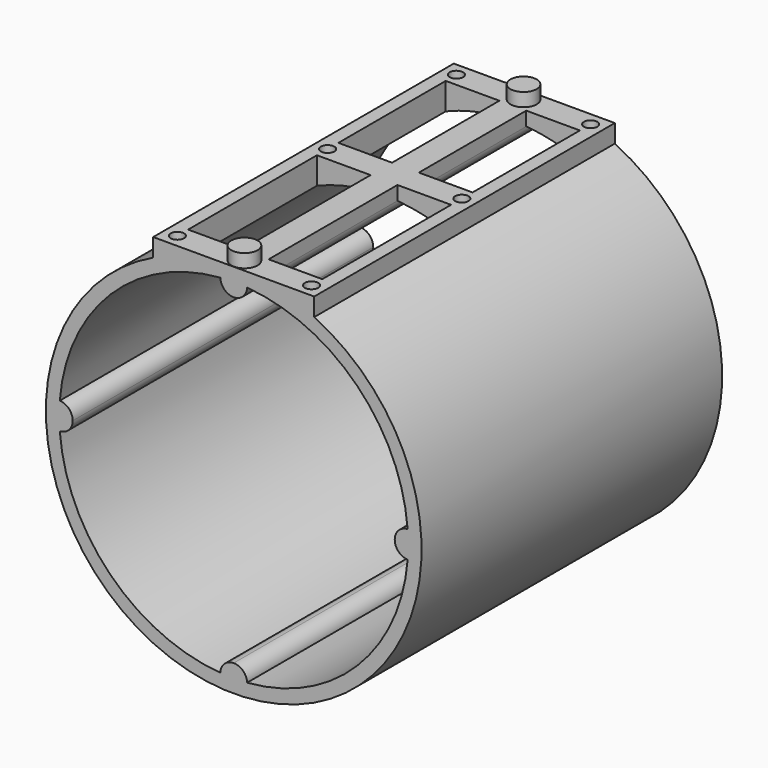
from build123d import *

# Parameters (mm, degrees)
F1_DEPTH = 177.8
F4_DEPTH = 177.801
F5_W     = 25.4
F5_H     = 76.2
F5_H_2   = 63.5
F6_DEPTH = 25.4
F7_R     = 3.175
F8_DEPTH = 25.4
F7_R_2   = 6.223
F9_DEPTH = 6.35


# Not quite as in the source:
# - a feature names something its author has since deleted; it is built from what else it names


with BuildPart() as f1:
    # F0 (on Front) → F1 (new body)
    with BuildSketch(Plane.XZ):
        with BuildLine():
            ThreePointArc((-38.1, 80.3218525683), (-47.519048812, -75.1342132454), (88.9, 0))
            ThreePointArc((88.9, 0), (75.1342132454, 47.519048812), (38.1, 80.3218525683))
            ThreePointArc((38.1, 80.3218525683), (19.5268700344, 86.7289533354), (0, 88.9))
            ThreePointArc((0, 88.9), (-19.5268700344, 86.7289533354), (-38.1, 80.3218525683))
        make_face()
        with BuildLine():
            ThreePointArc((0, 88.9), (19.5268700344, 86.7289533354), (38.1, 80.3218525683))
            Line((38.1, 80.3218525683), (38.1, 88.9))
            Line((38.1, 88.9), (0, 88.9))
        make_face()
        with BuildLine():
            Line((-38.1, 88.9), (-38.1, 80.3218525683))
            ThreePointArc((-38.1, 80.3218525683), (-19.5268700344, 86.7289533354), (0, 88.9))
            Line((0, 88.9), (-38.1, 88.9))
        make_face()
    extrude(amount=-F1_DEPTH)

    # F3 (on face) → F4 (cut, through all)
    with BuildSketch(Plane.XZ):
        with BuildLine():
            Line((-76.2, 0), (0, 0))
            Line((0, 0), (0, 76.2))
            ThreePointArc((0, 76.2), (-4.4029328075, 77.974338005), (-6.3453015162, 82.3057692308))
            ThreePointArc((-6.3453015162, 82.3057692308), (-58.3716647869, 58.3716647869), (-82.3057692308, 6.3453015162))
            ThreePointArc((-82.3057692308, 6.3453015162), (-77.974338005, 4.4029328075), (-76.2, 0))
        make_face()
        with BuildLine():
            Line((0, -76.2), (0, 0))
            Line((0, 0), (-76.2, 0))
            ThreePointArc((-76.2, 0), (-77.974338005, -4.4029328075), (-82.3057692308, -6.3453015162))
            ThreePointArc((-82.3057692308, -6.3453015162), (-58.3716647869, -58.3716647869), (-6.3453015162, -82.3057692308))
            ThreePointArc((-6.3453015162, -82.3057692308), (-4.4029328075, -77.974338005), (0, -76.2))
        make_face()
        with BuildLine():
            Line((0, 76.2), (0, 0))
            Line((0, 0), (76.2, 0))
            ThreePointArc((76.2, 0), (77.974338005, 4.4029328075), (82.3057692308, 6.3453015162))
            ThreePointArc((82.3057692308, 6.3453015162), (58.3716647869, 58.3716647869), (6.3453015162, 82.3057692308))
            ThreePointArc((6.3453015162, 82.3057692308), (4.4029328075, 77.974338005), (0, 76.2))
        make_face()
        with BuildLine():
            Line((76.2, 0), (0, 0))
            Line((0, 0), (0, -76.2))
            ThreePointArc((0, -76.2), (4.4029328075, -77.974338005), (6.3453015162, -82.3057692308))
            ThreePointArc((6.3453015162, -82.3057692308), (58.3716647869, -58.3716647869), (82.3057692308, -6.3453015162))
            ThreePointArc((82.3057692308, -6.3453015162), (77.974338005, -4.4029328075), (76.2, 0))
        make_face()
    extrude(amount=-F4_DEPTH, mode=Mode.SUBTRACT)

    # F5 (on face) → F6 (cut)
    with BuildSketch(Plane.XY.offset(88.9)):
        with Locations((-19.05, 50.8)):
            Rectangle(F5_W, F5_H)
        with Locations((19.05, 50.8)):
            Rectangle(F5_W, F5_H)
        with Locations((19.05, 133.35)):
            Rectangle(F5_W, F5_H_2)
        with Locations((-19.05, 133.35)):
            Rectangle(F5_W, F5_H_2)
    extrude(amount=-F6_DEPTH, mode=Mode.SUBTRACT)

    # F7 (on face) → F8 (cut)
    with BuildSketch(Plane.XY.offset(88.9)):
        with Locations((-31.75, 95.25)):
            Circle(F7_R)
        with Locations((-31.75, 171.45)):
            Circle(F7_R)
        with Locations((31.75, 171.45)):
            Circle(F7_R)
        with Locations((31.75, 95.25)):
            Circle(F7_R)
        with Locations((31.75, 6.35)):
            Circle(F7_R)
        with Locations((-31.75, 6.35)):
            Circle(F7_R)
    extrude(amount=-F8_DEPTH, mode=Mode.SUBTRACT)

    # F7 (on face) → F9 (join)
    with BuildSketch(Plane.XY.offset(88.9)):
        with Locations((0, 171.45)):
            Circle(F7_R_2)
        with Locations((0, 6.35)):
            Circle(F7_R_2)
    extrude(amount=F9_DEPTH)


solid = f1.part
